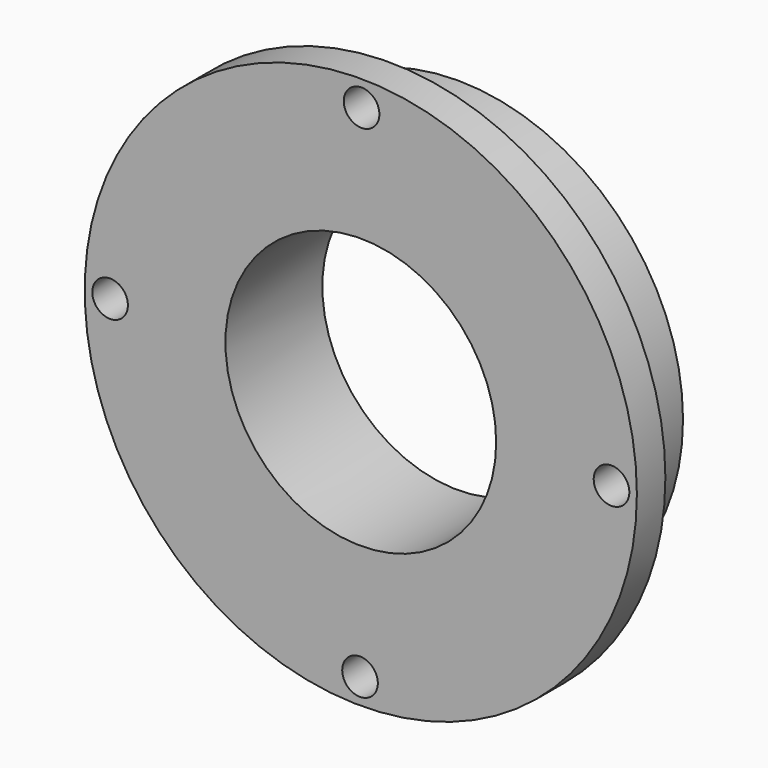
from build123d import *

# Parameters (mm, degrees)
F0_R     = 12.65
F1_DEPTH = 4.8
F2_R     = 15.5
F2_R_2   = 12.65
F3_DEPTH = 2
F4_R     = 1
F5_DEPTH = 2
F6_R     = 7.6
F7_DEPTH = 7


# Not quite as in the source:
# - a feature names something its author has since deleted; it is built from what else it names


with BuildPart() as f1:
    # F0 (on Front) → F1 (new body)
    with BuildSketch(Plane.XZ):
        Circle(F0_R)
    extrude(amount=F1_DEPTH)

    # F2 (on face) → F3 (join)
    with BuildSketch(Plane.XZ.offset(4.8)):
        Circle(F2_R)
        Circle(F2_R_2, mode=Mode.SUBTRACT)
        Circle(F2_R_2)
    extrude(amount=F3_DEPTH)

    # F4 (on face) → F5 (cut)
    with BuildSketch(Plane(origin=(0, -4.8, 0), x_dir=(-1, 0, 0), z_dir=(0, 1, 0))):
        with Locations((-0.0435703545, 14.074932562)):
            Circle(F4_R)
        with Locations((-14.074932562, -0.0435703545)):
            Circle(F4_R)
        with Locations((0.0435703545, -14.074932562)):
            Circle(F4_R)
        with Locations((14.074932562, 0.0435703545)):
            Circle(F4_R)
    extrude(amount=-F5_DEPTH, mode=Mode.SUBTRACT)

    # F6 (on face) → F7 (cut)
    with BuildSketch(Plane.XZ.offset(6.8)):
        Circle(F6_R)
    extrude(amount=-F7_DEPTH, mode=Mode.SUBTRACT)


solid = f1.part
